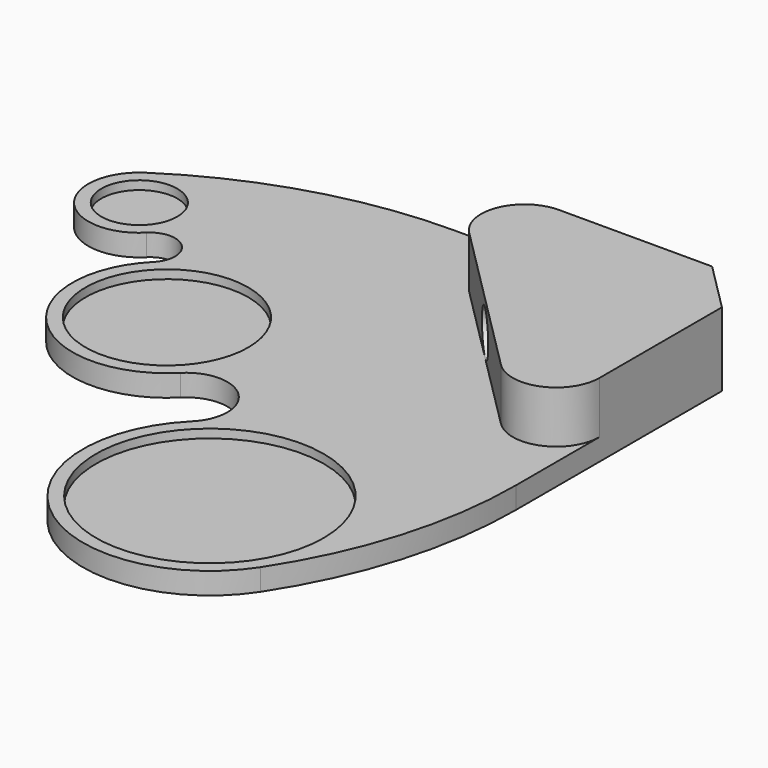
from build123d import *

# Parameters (mm, degrees)
F1_DEPTH     = 5
F2_R         = 8.75
F2_R_2       = 18.75
F2_R_3       = 26.25
F3_DEPTH     = 2
F5_DEPTH     = 12
F6_R         = 3.175
F7_DEPTH     = 183.6597451804
F8_R         = 5.08
F9_DEPTH     = 30
F10_S5_R     = 5.08
F10_T6_DEPTH = 9
F11_R        = 10


# Not quite as in the source:
# - a fillet or chamfer that OpenCascade refuses, or shapes differently, is made with other operations: its cross-section is extruded or revolved along the edge and cut away or added


with BuildPart() as f1:
    # F0 (on Top) → F1 (new body)
    with BuildSketch(Plane.XY):
        with BuildLine():
            ThreePointArc((89.2893218813, 160), (59.2982241526, 155.6212032378), (31.8110246399, 142.8503901468))
            ThreePointArc((31.8110246399, 142.8503901468), (29.1326558006, 125.6088436513), (46.5579786953, 124.7129043596))
            ThreePointArc((46.5579786953, 124.7129043596), (54.6897066789, 124.7129043596), (54.6897066789, 116.581176376))
            ThreePointArc((54.6897066789, 116.581176376), (54.6897066789, 85.8220313944), (85.4488516605, 85.8220313944))
            ThreePointArc((85.4488516605, 85.8220313944), (98.8838805031, 85.8220313944), (98.8838805031, 72.3870025518))
            ThreePointArc((98.8838805031, 72.3870025518), (101.1313528665, 28.995133397), (144.0588384666, 35.7134978428))
            ThreePointArc((144.0588384666, 35.7134978428), (155.9302038799, 61.3407550467), (160, 89.2893218813))
            Line((160, 89.2893218813), (160, 148.686291501))
            Line((160, 148.686291501), (148.686291501, 160))
            Line((148.686291501, 160), (89.2893218813, 160))
        make_face()
    extrude(amount=-F1_DEPTH)

    # F2 (on Top) → F3 (cut)
    with BuildSketch(Plane.XY):
        with Locations((38.2494740163, 133.0214090386)):
            Circle(F2_R)
        with Locations((70.0692791697, 101.2016038852)):
            Circle(F2_R_2)
        with Locations((119.5667538528, 51.7041292021)):
            Circle(F2_R_3)
    extrude(amount=-F3_DEPTH, mode=Mode.SUBTRACT)

    # F4 (on Top) → F5 (join)
    with BuildSketch(Plane.XY):
        Polygon((160, 148.686291501), (148.686291501, 160), (89.2893218813, 160), (160, 89.2893218813), align=None)
    extrude(amount=F5_DEPTH)

    # F6 (on face) → F7 (cut, through all)
    with BuildSketch(Plane(origin=(154.3431457505, 154.3431457505, 0), x_dir=(-0.7071067812, 0.7071067812, 0), z_dir=(0.7071067812, 0.7071067812, 0))):
        with Locations((0, 5.08)):
            Circle(F6_R)
    extrude(amount=-F7_DEPTH, mode=Mode.SUBTRACT)

    # F8 (on face) → F9 (cut)
    with BuildSketch(Plane(origin=(124.6446609407, 124.6446609407, 0), x_dir=(0.7071067812, -0.7071067812, 0), z_dir=(-0.7071067812, -0.7071067812, 0))):
        with Locations((0, 5.08)):
            Circle(F8_R)
    extrude(amount=-F9_DEPTH, mode=Mode.SUBTRACT)

    # F10: chamfer of 2 on 1 edges, made by hand


with BuildPart() as f10_tool2:
    # F10_s3 → F10_t4 (revolve)
    with BuildSketch(Plane.XY.offset(5.08)):
        Polygon((145.0270139084, 149.5171419689), (142.1985867836, 149.5171419689), (143.612800346, 148.1029284065), align=None)
    revolve(axis=Axis((145.8578643763, 145.8578643763, 5.08), (0.7071067812, 0.7071067812, 0)))

    # F10_s5 → F10_t6 (intersect, symmetric)
    with BuildSketch(Plane(origin=(145.8761289588, 145.8761289588, 0), x_dir=(0, 0, 1), z_dir=(-0.7071067812, -0.7071067812, 0))):
        with Locations((5.08, 0)):
            Circle(F10_S5_R)
    extrude(amount=F10_T6_DEPTH, both=True, mode=Mode.INTERSECT)


with BuildPart() as f1_1:
    add(f1.part)

    # F10_t1: cut F10_tool2
    add(f10_tool2.part, mode=Mode.SUBTRACT)

    # F11
    f11_edges = [f1_1.edges().sort_by_distance(p)[0] for p in [
        (160, 89.289322, 6),
        (89.289322, 160, 6),
    ]]
    fillet(f11_edges, radius=F11_R)


solid = f1_1.part
